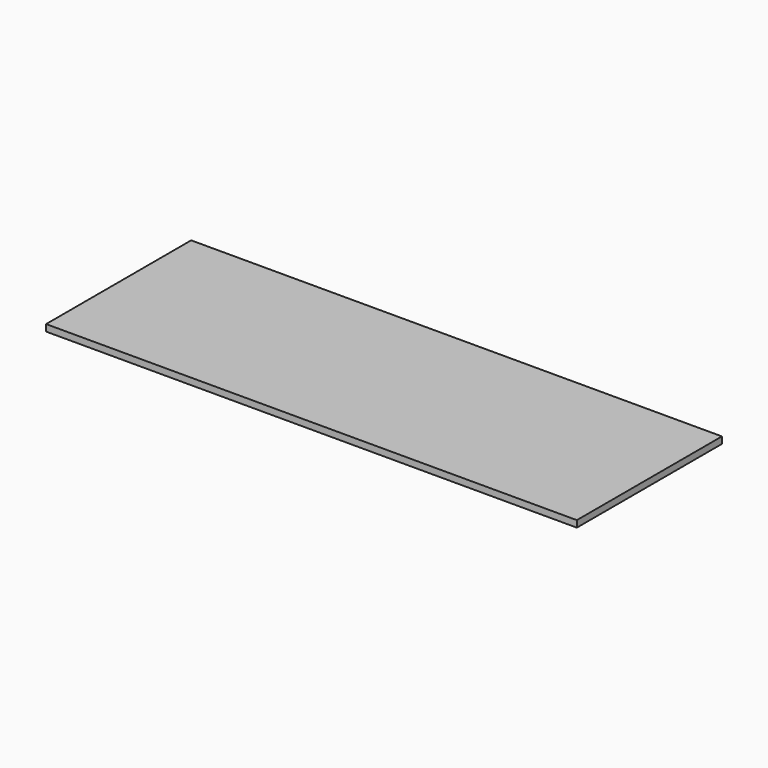
from build123d import *

# Parameters (mm, degrees)
F1_W     = 1524
F1_H     = 520.7
F2_DEPTH = 19.05


# Not quite as in the source:
# - a variable given as a bare number and used for a length is read in inches; the dataset says mm whatever the document's units were


with BuildPart() as f2:
    # F1 (on Top) → F2 (new body)
    with BuildSketch(Plane.XY):
        Rectangle(F1_W, F1_H)
    extrude(amount=-F2_DEPTH)


solid = f2.part
